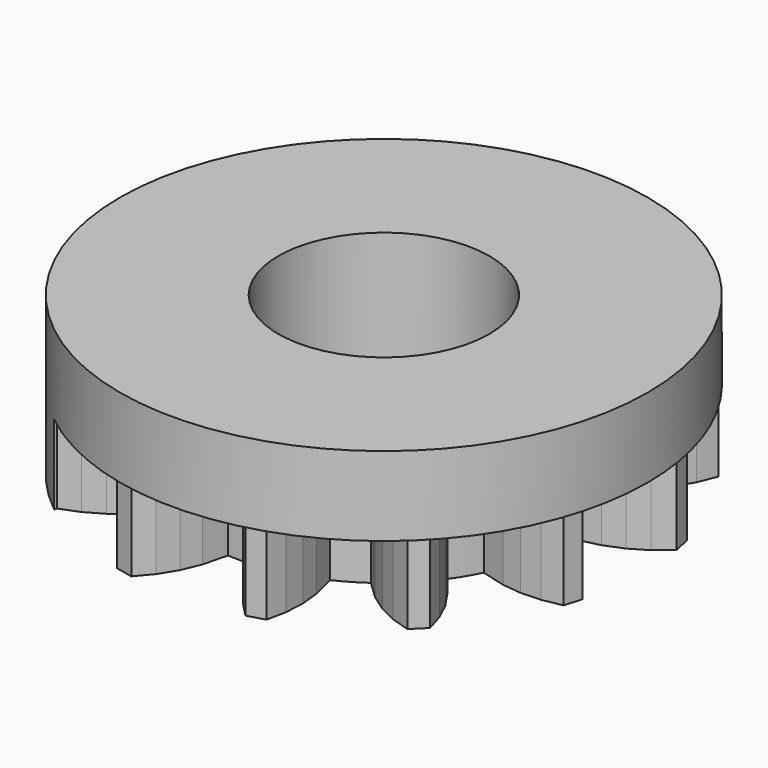
from build123d import *

# Parameters (mm, degrees)
F0_R     = 10
F0_R_2   = 4
F1_DEPTH = 3
F3_DEPTH = 25
F4_DEPTH = 3


# Not quite as in the source:
# - a feature names something its author has since deleted; it is built from what else it names


with BuildPart() as f1:
    # F0 (on Top) → F1 (new body)
    with BuildSketch(Plane.XY):
        with Locations((0, -55)):
            Circle(F0_R)
        with Locations((0, -55)):
            Circle(F0_R_2, mode=Mode.SUBTRACT)
    extrude(amount=-F1_DEPTH)

    # F2 (on face) → F3 (cut)
    with BuildSketch(Plane.XY):
        with BuildLine():
            ThreePointArc((6.918967171, -54.711004694), (6.9234916285, -54.8554708664), (6.925, -55))
            ThreePointArc((6.925, -55), (6.9091405252, -55.4684038892), (6.8616347427, -55.9346623229))
            Line((6.8616347427, -55.9346623229), (7.7608112736, -56.2391925528))
            Line((7.7608112736, -56.2391925528), (8.4266122732, -56.5844591584))
            Line((8.4266122732, -56.5844591584), (9.0325271812, -57.0264626926))
            Line((9.0325271812, -57.0264626926), (9.5646125465, -57.5550316702))
            Line((9.5646125465, -57.5550316702), (9.3682753061, -58.2008464176))
            Line((9.3682753061, -58.2008464176), (8.6320298332, -58.3438240508))
            Line((8.6320298332, -58.3438240508), (7.8826287699, -58.373791473))
            Line((7.8826287699, -58.373791473), (7.1373175032, -58.2900590671))
            Line((7.1373175032, -58.2900590671), (6.2207936805, -58.0425895196))
            ThreePointArc((6.2207936805, -58.0425895196), (5.9273034064, -58.5808796864), (5.5873528695, -59.0911016746))
            Line((5.5873528695, -59.0911016746), (6.2328020031, -59.7872715608))
            Line((6.2328020031, -59.7872715608), (6.6536597658, -60.4080603684))
            Line((6.6536597658, -60.4080603684), (6.9757740672, -61.0853656001))
            Line((6.9757740672, -61.0853656001), (7.1917323401, -61.8036009545))
            Line((7.1917323401, -61.8036009545), (6.7114037747, -62.2778471661))
            Line((6.7114037747, -62.2778471661), (5.9959787098, -62.0527539043))
            Line((5.9959787098, -62.0527539043), (5.322833198, -61.722034809))
            Line((5.322833198, -61.722034809), (4.7074578164, -61.2933004628))
            Line((4.7074578164, -61.2933004628), (4.0195694603, -60.6390323951))
            ThreePointArc((4.0195694603, -60.6390323951), (3.5050568866, -60.9724535345), (2.9630704597, -61.2590605087))
            Line((2.9630704597, -61.2590605087), (3.1988405858, -62.1786634351))
            Line((3.1988405858, -62.1786634351), (3.2730686388, -62.9249811932))
            Line((3.2730686388, -62.9249811932), (3.2335539791, -63.673939531))
            Line((3.2335539791, -63.673939531), (3.0812059272, -64.4083032495))
            Line((3.0812059272, -64.4083032495), (2.4329416781, -64.5963948851))
            Line((2.4329416781, -64.5963948851), (1.9111960197, -64.0576171313))
            Line((1.9111960197, -64.0576171313), (1.476949591, -63.4461189391))
            Line((1.476949591, -63.4461189391), (1.1401953689, -62.7759722433))
            Line((1.1401953689, -62.7759722433), (0.8471481357, -61.8729880719))
            ThreePointArc((0.8471481357, -61.8729880719), (0.2359283481, -61.9209799028), (-0.3771407279, -61.9147226894))
            Line((-0.3771407279, -61.9147226894), (-0.6080157262, -62.8355667749))
            Line((-0.6080157262, -62.8355667749), (-0.898352157, -63.5270902792))
            Line((-0.898352157, -63.5270902792), (-1.2899483564, -64.1667405091))
            Line((-1.2899483564, -64.1667405091), (-1.773792824, -64.7397976887))
            Line((-1.773792824, -64.7397976887), (-2.4333609662, -64.5962885747))
            Line((-2.4333609662, -64.5962885747), (-2.6353644947, -63.8740042993))
            Line((-2.6353644947, -63.8740042993), (-2.7257904358, -63.1294754891))
            Line((-2.7257904358, -63.1294754891), (-2.7025578872, -62.3798354097))
            Line((-2.7025578872, -62.3798354097), (-2.5299587465, -61.4463116385))
            ThreePointArc((-2.5299587465, -61.4463116385), (-3.0902045366, -61.1972785093), (-3.6262282301, -60.8996689588))
            Line((-3.6262282301, -60.8996689588), (-4.267964983, -61.5992624369))
            Line((-4.267964983, -61.5992624369), (-4.852715623, -62.0689077169))
            Line((-4.852715623, -62.0689077169), (-5.5017769863, -62.4446993436))
            Line((-5.5017769863, -62.4446993436), (-6.2002127258, -62.7179895151))
            Line((-6.2002127258, -62.7179895151), (-6.2293167628, -62.8227624704))
            ThreePointArc((-6.2293167628, -62.8227624704), (4.3420520709, -64.0081398643), (10, -55))
            ThreePointArc((10, -55), (8.9702732091, -50.5802490393), (6.093160289, -47.0707252733))
            Line((6.093160289, -47.0707252733), (4.5292177041, -49.7615067062))
            Line((4.5292177041, -49.7615067062), (5.2752674988, -49.1744234085))
            Line((5.2752674988, -49.1744234085), (5.9280342708, -48.8051057384))
            Line((5.9280342708, -48.8051057384), (6.6291535281, -48.5387755166))
            Line((6.6291535281, -48.5387755166), (7.3624909556, -48.3815615944))
            Line((7.3624909556, -48.3815615944), (7.7963725922, -48.8986415935))
            Line((7.7963725922, -48.8986415935), (7.5142043948, -49.5935380667))
            Line((7.5142043948, -49.5935380667), (7.1301722462, -50.2377579894))
            Line((7.1301722462, -50.2377579894), (6.653113581, -50.8164764269))
            Line((6.653113581, -50.8164764269), (5.9453992104, -51.4492461041))
            ThreePointArc((5.9453992104, -51.4492461041), (6.2361540084, -51.9890187341), (6.4780276654, -52.552392481))
            Line((6.4780276654, -52.552392481), (7.4136750809, -52.3917033141))
            Line((7.4136750809, -52.3917033141), (8.1635503464, -52.3780253684))
            Line((8.1635503464, -52.3780253684), (8.9068663995, -52.4779315504))
            Line((8.9068663995, -52.4779315504), (9.6265178829, -52.6891227965))
            Line((9.6265178829, -52.6891227965), (9.7616104212, -53.350466131))
            Line((9.7616104212, -53.350466131), (9.1824341074, -53.8269688042))
            Line((9.1824341074, -53.8269688042), (8.5378456767, -54.2103820995))
            Line((8.5378456767, -54.2103820995), (7.8426785438, -54.4918828231))
            Line((7.8426785438, -54.4918828231), (6.918967171, -54.711004694))
        make_face()
    extrude(amount=-F3_DEPTH, mode=Mode.SUBTRACT)

    # F0 (on Top) → F4 (join)
    with BuildSketch(Plane.XY):
        with Locations((0, -55)):
            Circle(F0_R)
        with Locations((0, -55)):
            Circle(F0_R_2, mode=Mode.SUBTRACT)
    extrude(amount=F4_DEPTH)


solid = f1.part
